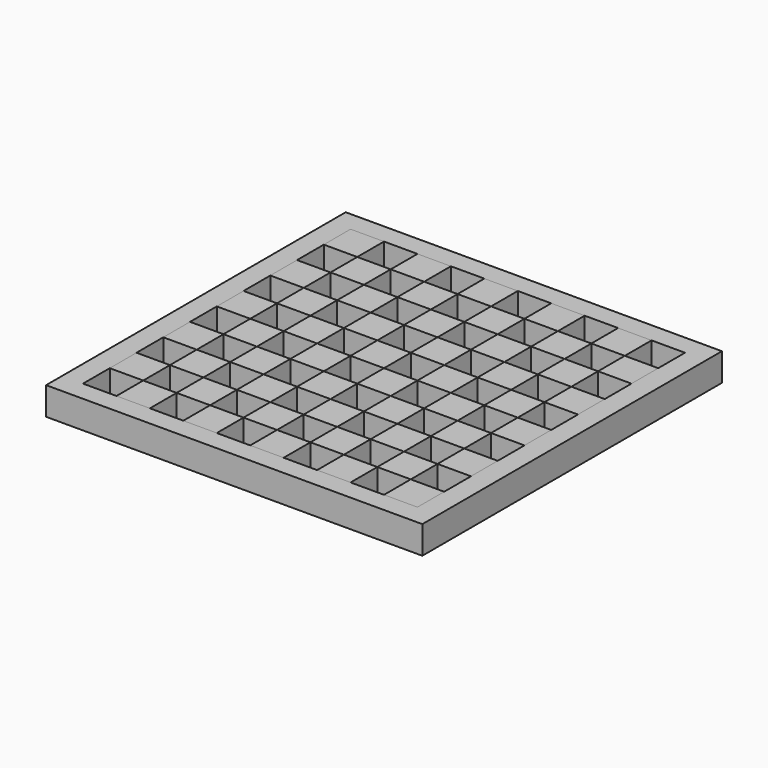
from build123d import *

# Parameters (mm, degrees)
F0_W     = 342.9
F0_H     = 341.3125
F0_W_2   = 304.8
F0_H_2   = 304.8
F2_DEPTH = 25.4
F1_W     = 30.48
F1_H     = 30.48
F3_DEPTH = 25.4


# Not quite as in the source:
# - ends of sketch curves that miss each other by under 0.0002 mm in the source are joined


with BuildPart() as f2:
    # F0 (on Top) → F2 (new body)
    with BuildSketch(Plane.XY):
        Rectangle(F0_W, F0_H)
        Rectangle(F0_W_2, F0_H_2, mode=Mode.SUBTRACT)
    extrude(amount=-F2_DEPTH)


with BuildPart() as f3:
    # F1 (on face) → F3 (new body)
    with BuildSketch(Plane.XY):
        with Locations((-137.16, 137.16)):
            Rectangle(F1_W, F1_H)
    extrude(amount=-F3_DEPTH)


with BuildPart() as f3b:
    # F1 (on face) → F3, piece 2 (new body)
    with BuildSketch(Plane.XY):
        with Locations((-106.68, 106.68)):
            Rectangle(F1_W, F1_H)
    extrude(amount=-F3_DEPTH)


with BuildPart() as f3c:
    # F1 (on face) → F3, piece 3 (new body)
    with BuildSketch(Plane.XY):
        with Locations((-76.2, 137.16)):
            Rectangle(F1_W, F1_H)
    extrude(amount=-F3_DEPTH)


with BuildPart() as f3d:
    # F1 (on face) → F3, piece 4 (new body)
    with BuildSketch(Plane.XY):
        with Locations((-45.72, 106.68)):
            Rectangle(F1_W, F1_H)
    extrude(amount=-F3_DEPTH)


with BuildPart() as f3e:
    # F1 (on face) → F3, piece 5 (new body)
    with BuildSketch(Plane.XY):
        Polygon((0, 121.92), (0, 152.3999981165), (-30.48, 152.4), (-30.48, 121.92), align=None)
    extrude(amount=-F3_DEPTH)


with BuildPart() as f3f:
    # F1 (on face) → F3, piece 6 (new body)
    with BuildSketch(Plane.XY):
        with Locations((15.24, 106.68)):
            Rectangle(F1_W, F1_H)
    extrude(amount=-F3_DEPTH)


with BuildPart() as f3g:
    # F1 (on face) → F3, piece 7 (new body)
    with BuildSketch(Plane.XY):
        with Locations((45.72, 137.16)):
            Rectangle(F1_W, F1_H)
    extrude(amount=-F3_DEPTH)


with BuildPart() as f3h:
    # F1 (on face) → F3, piece 8 (new body)
    with BuildSketch(Plane.XY):
        with Locations((76.2, 106.68)):
            Rectangle(F1_W, F1_H)
    extrude(amount=-F3_DEPTH)


with BuildPart() as f3i:
    # F1 (on face) → F3, piece 9 (new body)
    with BuildSketch(Plane.XY):
        with Locations((106.68, 137.16)):
            Rectangle(F1_W, F1_H)
    extrude(amount=-F3_DEPTH)


with BuildPart() as f3j:
    # F1 (on face) → F3, piece 10 (new body)
    with BuildSketch(Plane.XY):
        with Locations((137.16, 106.68)):
            Rectangle(F1_W, F1_H)
    extrude(amount=-F3_DEPTH)


with BuildPart() as f3k:
    # F1 (on face) → F3, piece 11 (new body)
    with BuildSketch(Plane.XY):
        with Locations((-137.16, 76.2)):
            Rectangle(F1_W, F1_H)
    extrude(amount=-F3_DEPTH)


with BuildPart() as f3l:
    # F1 (on face) → F3, piece 12 (new body)
    with BuildSketch(Plane.XY):
        with Locations((-76.2, 76.2)):
            Rectangle(F1_W, F1_H)
    extrude(amount=-F3_DEPTH)


with BuildPart() as f3m:
    # F1 (on face) → F3, piece 13 (new body)
    with BuildSketch(Plane.XY):
        with Locations((-15.24, 76.2)):
            Rectangle(F1_W, F1_H)
    extrude(amount=-F3_DEPTH)


with BuildPart() as f3n:
    # F1 (on face) → F3, piece 14 (new body)
    with BuildSketch(Plane.XY):
        with Locations((45.72, 76.2)):
            Rectangle(F1_W, F1_H)
    extrude(amount=-F3_DEPTH)


with BuildPart() as f3o:
    # F1 (on face) → F3, piece 15 (new body)
    with BuildSketch(Plane.XY):
        with Locations((106.68, 76.2)):
            Rectangle(F1_W, F1_H)
    extrude(amount=-F3_DEPTH)


with BuildPart() as f3p:
    # F1 (on face) → F3, piece 16 (new body)
    with BuildSketch(Plane.XY):
        with Locations((137.16, 45.72)):
            Rectangle(F1_W, F1_H)
    extrude(amount=-F3_DEPTH)


with BuildPart() as f3q:
    # F1 (on face) → F3, piece 17 (new body)
    with BuildSketch(Plane.XY):
        with Locations((76.2, 45.72)):
            Rectangle(F1_W, F1_H)
    extrude(amount=-F3_DEPTH)


with BuildPart() as f3r:
    # F1 (on face) → F3, piece 18 (new body)
    with BuildSketch(Plane.XY):
        with Locations((15.24, 45.72)):
            Rectangle(F1_W, F1_H)
    extrude(amount=-F3_DEPTH)


with BuildPart() as f3s:
    # F1 (on face) → F3, piece 19 (new body)
    with BuildSketch(Plane.XY):
        with Locations((-45.72, 45.72)):
            Rectangle(F1_W, F1_H)
    extrude(amount=-F3_DEPTH)


with BuildPart() as f3t:
    # F1 (on face) → F3, piece 20 (new body)
    with BuildSketch(Plane.XY):
        with Locations((-106.68, 45.72)):
            Rectangle(F1_W, F1_H)
    extrude(amount=-F3_DEPTH)


with BuildPart() as f3u:
    # F1 (on face) → F3, piece 21 (new body)
    with BuildSketch(Plane.XY):
        with Locations((-137.16, 15.24)):
            Rectangle(F1_W, F1_H)
    extrude(amount=-F3_DEPTH)


with BuildPart() as f3v:
    # F1 (on face) → F3, piece 22 (new body)
    with BuildSketch(Plane.XY):
        with Locations((-76.2, 15.24)):
            Rectangle(F1_W, F1_H)
    extrude(amount=-F3_DEPTH)


with BuildPart() as f3w:
    # F1 (on face) → F3, piece 23 (new body)
    with BuildSketch(Plane.XY):
        with Locations((-15.24, 15.24)):
            Rectangle(F1_W, F1_H)
    extrude(amount=-F3_DEPTH)


with BuildPart() as f3x:
    # F1 (on face) → F3, piece 24 (new body)
    with BuildSketch(Plane.XY):
        with Locations((45.72, 15.24)):
            Rectangle(F1_W, F1_H)
    extrude(amount=-F3_DEPTH)


with BuildPart() as f3y:
    # F1 (on face) → F3, piece 25 (new body)
    with BuildSketch(Plane.XY):
        with Locations((106.68, 15.24)):
            Rectangle(F1_W, F1_H)
    extrude(amount=-F3_DEPTH)


with BuildPart() as f3z:
    # F1 (on face) → F3, piece 26 (new body)
    with BuildSketch(Plane.XY):
        with Locations((137.16, -15.24)):
            Rectangle(F1_W, F1_H)
    extrude(amount=-F3_DEPTH)


with BuildPart() as f3ba:
    # F1 (on face) → F3, piece 27 (new body)
    with BuildSketch(Plane.XY):
        with Locations((76.2, -15.24)):
            Rectangle(F1_W, F1_H)
    extrude(amount=-F3_DEPTH)


with BuildPart() as f3bb:
    # F1 (on face) → F3, piece 28 (new body)
    with BuildSketch(Plane.XY):
        with Locations((15.24, -15.24)):
            Rectangle(F1_W, F1_H)
    extrude(amount=-F3_DEPTH)


with BuildPart() as f3bc:
    # F1 (on face) → F3, piece 29 (new body)
    with BuildSketch(Plane.XY):
        with Locations((-45.72, -15.24)):
            Rectangle(F1_W, F1_H)
    extrude(amount=-F3_DEPTH)


with BuildPart() as f3bd:
    # F1 (on face) → F3, piece 30 (new body)
    with BuildSketch(Plane.XY):
        with Locations((-106.68, -15.24)):
            Rectangle(F1_W, F1_H)
    extrude(amount=-F3_DEPTH)


with BuildPart() as f3be:
    # F1 (on face) → F3, piece 31 (new body)
    with BuildSketch(Plane.XY):
        with Locations((-137.16, -45.72)):
            Rectangle(F1_W, F1_H)
    extrude(amount=-F3_DEPTH)


with BuildPart() as f3bf:
    # F1 (on face) → F3, piece 32 (new body)
    with BuildSketch(Plane.XY):
        with Locations((-76.2, -45.72)):
            Rectangle(F1_W, F1_H)
    extrude(amount=-F3_DEPTH)


with BuildPart() as f3bg:
    # F1 (on face) → F3, piece 33 (new body)
    with BuildSketch(Plane.XY):
        with Locations((-15.24, -45.72)):
            Rectangle(F1_W, F1_H)
    extrude(amount=-F3_DEPTH)


with BuildPart() as f3bh:
    # F1 (on face) → F3, piece 34 (new body)
    with BuildSketch(Plane.XY):
        with Locations((45.72, -45.72)):
            Rectangle(F1_W, F1_H)
    extrude(amount=-F3_DEPTH)


with BuildPart() as f3bi:
    # F1 (on face) → F3, piece 35 (new body)
    with BuildSketch(Plane.XY):
        with Locations((106.68, -45.72)):
            Rectangle(F1_W, F1_H)
    extrude(amount=-F3_DEPTH)


with BuildPart() as f3bj:
    # F1 (on face) → F3, piece 36 (new body)
    with BuildSketch(Plane.XY):
        with Locations((137.16, -76.2)):
            Rectangle(F1_W, F1_H)
    extrude(amount=-F3_DEPTH)


with BuildPart() as f3bk:
    # F1 (on face) → F3, piece 37 (new body)
    with BuildSketch(Plane.XY):
        with Locations((76.2, -76.2)):
            Rectangle(F1_W, F1_H)
    extrude(amount=-F3_DEPTH)


with BuildPart() as f3bl:
    # F1 (on face) → F3, piece 38 (new body)
    with BuildSketch(Plane.XY):
        with Locations((15.24, -76.2)):
            Rectangle(F1_W, F1_H)
    extrude(amount=-F3_DEPTH)


with BuildPart() as f3bm:
    # F1 (on face) → F3, piece 39 (new body)
    with BuildSketch(Plane.XY):
        with Locations((-45.72, -76.2)):
            Rectangle(F1_W, F1_H)
    extrude(amount=-F3_DEPTH)


with BuildPart() as f3bn:
    # F1 (on face) → F3, piece 40 (new body)
    with BuildSketch(Plane.XY):
        with Locations((-106.68, -76.2)):
            Rectangle(F1_W, F1_H)
    extrude(amount=-F3_DEPTH)


with BuildPart() as f3bo:
    # F1 (on face) → F3, piece 41 (new body)
    with BuildSketch(Plane.XY):
        with Locations((-137.16, -106.68)):
            Rectangle(F1_W, F1_H)
    extrude(amount=-F3_DEPTH)


with BuildPart() as f3bp:
    # F1 (on face) → F3, piece 42 (new body)
    with BuildSketch(Plane.XY):
        with Locations((-76.2, -106.68)):
            Rectangle(F1_W, F1_H)
    extrude(amount=-F3_DEPTH)


with BuildPart() as f3bq:
    # F1 (on face) → F3, piece 43 (new body)
    with BuildSketch(Plane.XY):
        with Locations((-15.24, -106.68)):
            Rectangle(F1_W, F1_H)
    extrude(amount=-F3_DEPTH)


with BuildPart() as f3br:
    # F1 (on face) → F3, piece 44 (new body)
    with BuildSketch(Plane.XY):
        with Locations((45.72, -106.68)):
            Rectangle(F1_W, F1_H)
    extrude(amount=-F3_DEPTH)


with BuildPart() as f3bs:
    # F1 (on face) → F3, piece 45 (new body)
    with BuildSketch(Plane.XY):
        with Locations((106.68, -106.68)):
            Rectangle(F1_W, F1_H)
    extrude(amount=-F3_DEPTH)


with BuildPart() as f3bt:
    # F1 (on face) → F3, piece 46 (new body)
    with BuildSketch(Plane.XY):
        with Locations((137.16, -137.16)):
            Rectangle(F1_W, F1_H)
    extrude(amount=-F3_DEPTH)


with BuildPart() as f3bu:
    # F1 (on face) → F3, piece 47 (new body)
    with BuildSketch(Plane.XY):
        with Locations((76.2, -137.16)):
            Rectangle(F1_W, F1_H)
    extrude(amount=-F3_DEPTH)


with BuildPart() as f3bv:
    # F1 (on face) → F3, piece 48 (new body)
    with BuildSketch(Plane.XY):
        Polygon((30.48, -152.4), (30.48, -121.92), (0, -121.92), (0, -152.4000018835), align=None)
    extrude(amount=-F3_DEPTH)


with BuildPart() as f3bw:
    # F1 (on face) → F3, piece 49 (new body)
    with BuildSketch(Plane.XY):
        with Locations((-45.72, -137.16)):
            Rectangle(F1_W, F1_H)
    extrude(amount=-F3_DEPTH)


with BuildPart() as f3bx:
    # F1 (on face) → F3, piece 50 (new body)
    with BuildSketch(Plane.XY):
        with Locations((-106.68, -137.16)):
            Rectangle(F1_W, F1_H)
    extrude(amount=-F3_DEPTH)


solid = Compound([f2.part, f3.part, f3b.part, f3c.part, f3d.part, f3e.part, f3f.part, f3g.part, f3h.part, f3i.part, f3j.part, f3k.part, f3l.part, f3m.part, f3n.part, f3o.part, f3p.part, f3q.part, f3r.part, f3s.part, f3t.part, f3u.part, f3v.part, f3w.part, f3x.part, f3y.part, f3z.part, f3ba.part, f3bb.part, f3bc.part, f3bd.part, f3be.part, f3bf.part, f3bg.part, f3bh.part, f3bi.part, f3bj.part, f3bk.part, f3bl.part, f3bm.part, f3bn.part, f3bo.part, f3bp.part, f3bq.part, f3br.part, f3bs.part, f3bt.part, f3bu.part, f3bv.part, f3bw.part, f3bx.part])
